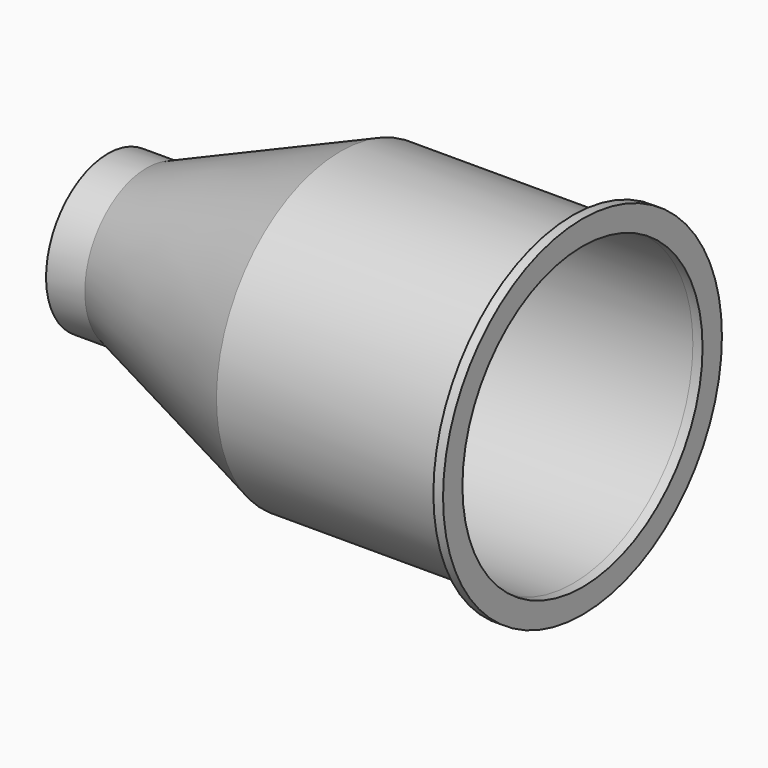
from build123d import *
from build123d import SkipClean  # not in build123d's __all__

# Parameters (mm, degrees)
F2_R     = 57.15
F2_R_2   = 49.2125
F3_DEPTH = 3.175


# Not quite as in the source:
# - a feature of the source that left no trace in its solid (it failed there, or was rolled back) is left out


with BuildPart() as f1:
    # F0 (on Front) → F1 (revolve)
    with BuildSketch(Plane.XZ):
        Polygon((152.4, 50.8), (76.2, 50.8), (12.7, 25.4), (0, 25.4), (0, 3.175), (1.5875, 3.175), (1.5875, 23.8125), (13.0057245657, 23.8125), (76.5057245657, 49.2125), (152.4, 49.2125), align=None)
    revolve(axis=Axis((76.2, 0, 0), (1, 0, 0)))

    # F2 (on face) → F3 (join)
    with BuildSketch(Plane.YZ.offset(152.4)):
        Circle(F2_R)
        Circle(F2_R_2, mode=Mode.SUBTRACT)
    with SkipClean():  # cleaning this boolean's faces spoils the solid; the shape is the same uncleaned
        extrude(amount=F3_DEPTH)


solid = f1.part
